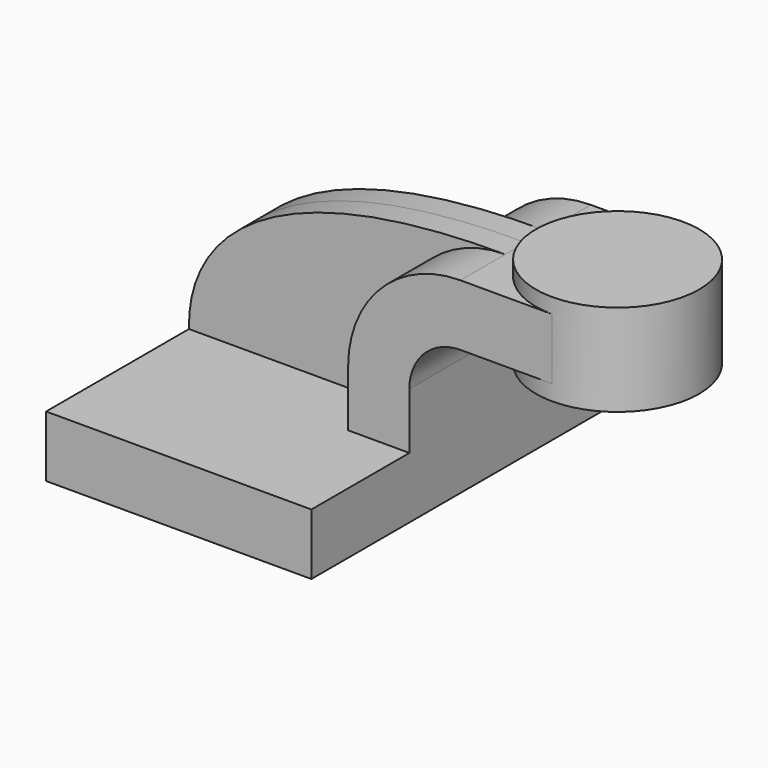
from build123d import *

# Parameters (mm, degrees)
F1_DEPTH = 63.5
F0_W     = 25.4
F0_H     = 19.05
F2_DEPTH = 25.4
F3_DEPTH = 7.9375


with BuildPart() as f1:
    # F0 (on Front) → F1 (new body, symmetric)
    with BuildSketch(Plane.XZ):
        Polygon((-41.275, 9.525), (-41.275, -9.525), (41.275, -9.525), (41.275, 9.525), (22.225, 9.525), align=None)
    extrude(amount=F1_DEPTH, both=True)

    # F0 (on Front) → F2 (join, symmetric)
    with BuildSketch(Plane.XZ):
        with BuildLine():
            Line((22.225, 9.525), (41.275, 9.525))
            Line((41.275, 9.525), (41.275, 27.051))
            ThreePointArc((41.275, 27.051), (45.9246798487, 38.2763201513), (57.15, 42.926))
            Line((57.15, 42.926), (60.325, 42.926))
            Line((60.325, 42.926), (60.325, 61.976))
            Line((60.325, 61.976), (57.15, 61.976))
            ThreePointArc((57.15, 61.976), (32.4542956671, 51.7467043329), (22.225, 27.051))
            Line((22.225, 27.051), (22.225, 9.525))
        make_face()
        with Locations((73.025, 52.451)):
            Rectangle(F0_W, F0_H)
    extrude(amount=F2_DEPTH, both=True)

    # F0 (on Front) → F3 (join, symmetric)
    with BuildSketch(Plane.XZ):
        with BuildLine():
            add(Edge.make_bspline(
                [(-41.275, 9.525), (-41.8424867094, 37.764005363), (-14.1566935927, 62.2859746218), (57.15, 61.976)],
                knots=[0, 0, 0, 0, 111.5284180198, 111.5284180198, 111.5284180198, 111.5284180198], degree=3))
            Line((-41.275, 9.525), (22.225, 9.525))
            Line((22.225, 9.525), (22.225, 27.051))
            ThreePointArc((22.225, 27.051), (32.4542956671, 51.7467043329), (57.15, 61.976))
        make_face()
    extrude(amount=F3_DEPTH, both=True)

    # F0 (on Front) → F4 (revolve)
    with BuildSketch(Plane.XZ):
        Polygon((85.725, 66.675), (85.725, 61.976), (85.725, 42.926), (85.725, 38.1), (111.125, 38.1), (111.125, 66.675), align=None)
    revolve(axis=Axis((85.725, 0, 52.3875), (0, 0, 1)))


solid = f1.part
